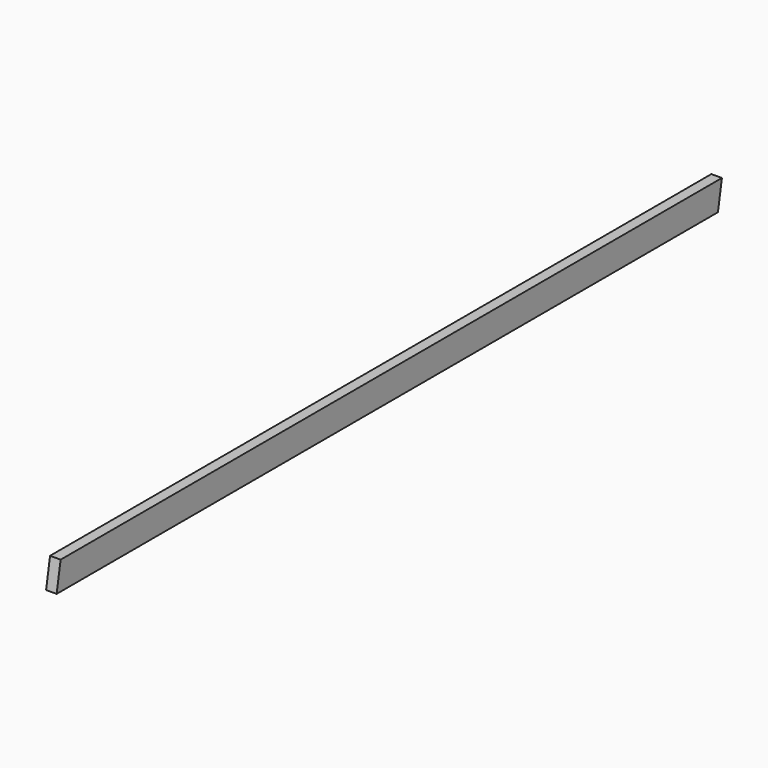
from build123d import *

# Parameters (mm, degrees)
F0_W     = 19.05
F0_H     = 1500.7336
F1_DEPTH = 50.8
F3_DEPTH = 19.051


# Not quite as in the source:
# - a feature names something its author has since deleted; it is built from what else it names


with BuildPart() as f1:
    # F0 (on Top) → F1 (new body)
    with BuildSketch(Plane.XY):
        with Locations((9.525, 750.3668)):
            Rectangle(F0_W, F0_H)
    extrude(amount=F1_DEPTH)

    # F2 (on face) → F3 (cut, through all)
    with BuildSketch(Plane.YZ.offset(19.05)):
        Polygon((8.95741062, 50.8), (0, 50.8), (0, 0), align=None)
        Polygon((1500.7336, 50.8), (1491.77618938, 0), (1500.7336, 0), align=None)
    extrude(amount=-F3_DEPTH, mode=Mode.SUBTRACT)


solid = f1.part
